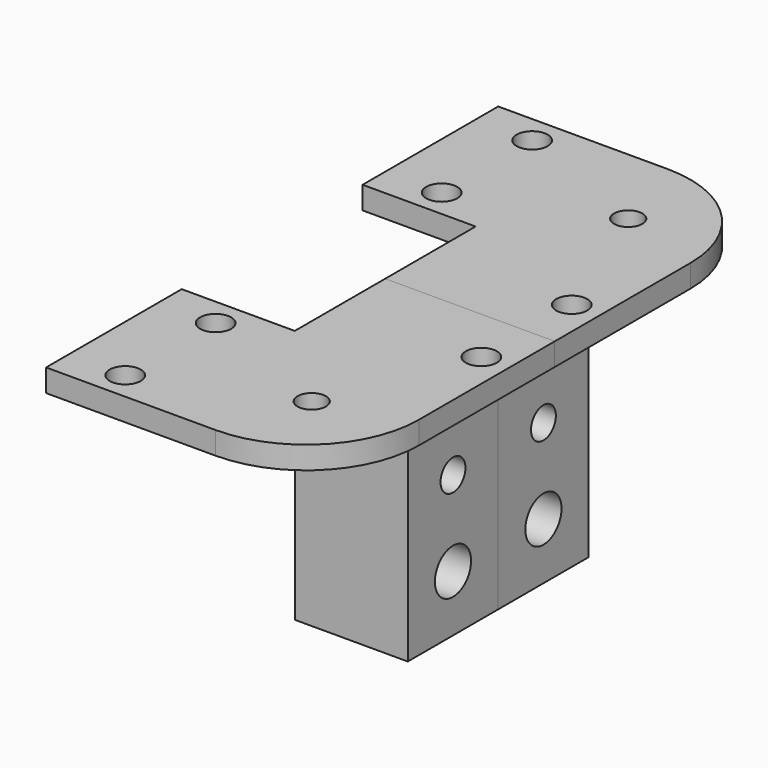
from build123d import *

# Parameters (mm, degrees)
F0_W      = 30
F0_H      = 30
F1_DEPTH  = 2
F2_DEPTH  = 20
F3_R      = 2.75
F4_DEPTH  = 4.001
F5_W      = 20
F5_H      = 45
F6_DEPTH  = 20
F7_DEPTH  = 20
F8_R      = 4
F8_R_2    = 2.75
F9_DEPTH  = 40.001
F10_R     = 2.75
F11_DEPTH = 4.001
F12_R     = 2.5
F13_DEPTH = 45.001
F14_R     = 20


with BuildPart() as f1:
    # F0 (on Top) → F1 (new body, symmetric)
    with BuildSketch(Plane.XY):
        Rectangle(F0_W, F0_H)
    extrude(amount=F1_DEPTH, both=True)

    # F2 (add): a face of the model
    f2_faces = [f1.faces().sort_by_distance(p)[0] for p in [
        (-15, 0, 0),
    ]]
    extrude(f2_faces, amount=F2_DEPTH)

    # F3 (on face) → F4 (cut, through all)
    with BuildSketch(Plane.XY.offset(2)):
        with Locations((-25, 10)):
            Circle(F3_R)
        with Locations((-25, -10)):
            Circle(F3_R)
    extrude(amount=-F4_DEPTH, mode=Mode.SUBTRACT)

    # F5 (on face) → F6 (join)
    with BuildSketch(Plane(origin=(0, 15, 0), x_dir=(-1, 0, 0), z_dir=(0, 1, 0))):
        with Locations((5, -20.5)):
            Rectangle(F5_W, F5_H)
    extrude(amount=F6_DEPTH)

    # F7 (add, through all): a face of the model
    f7_faces = [f1.faces().sort_by_distance(p)[0] for p in [
        (10, 15, 0),
    ]]
    extrude(f7_faces, amount=F7_DEPTH)

    # F8 (on face) → F9 (cut, through all)
    with BuildSketch(Plane.YZ.offset(5)):
        with Locations((25, -33)):
            Circle(F8_R)
        with Locations((25, -18)):
            Circle(F8_R_2)
    extrude(amount=-F9_DEPTH, mode=Mode.SUBTRACT)

    # F10 (on face) → F11 (cut, through all)
    with BuildSketch(Plane(origin=(0, 0, -2), x_dir=(1, 0, 0), z_dir=(0, 0, -1))):
        with Locations((10, -25)):
            Circle(F10_R)
    extrude(amount=-F11_DEPTH, mode=Mode.SUBTRACT)

    # F12 (on face) → F13 (cut, through all)
    with BuildSketch(Plane.XY.offset(2)):
        Circle(F12_R)
    extrude(amount=-F13_DEPTH, mode=Mode.SUBTRACT)

    # F14
    f14_edges = [f1.edges().sort_by_distance(p)[0] for p in [
        (15, -15, 0),
    ]]
    fillet(f14_edges, radius=F14_R)


with BuildPart() as f15_1:
    # F15: instance of F1
    add(f1.part.mirror(Plane(origin=(-4.3617021277, 35, -19.6276595745), x_dir=(-1, 0, 0), z_dir=(0, 1, 0))))


solid = Compound([f1.part, f15_1.part])
